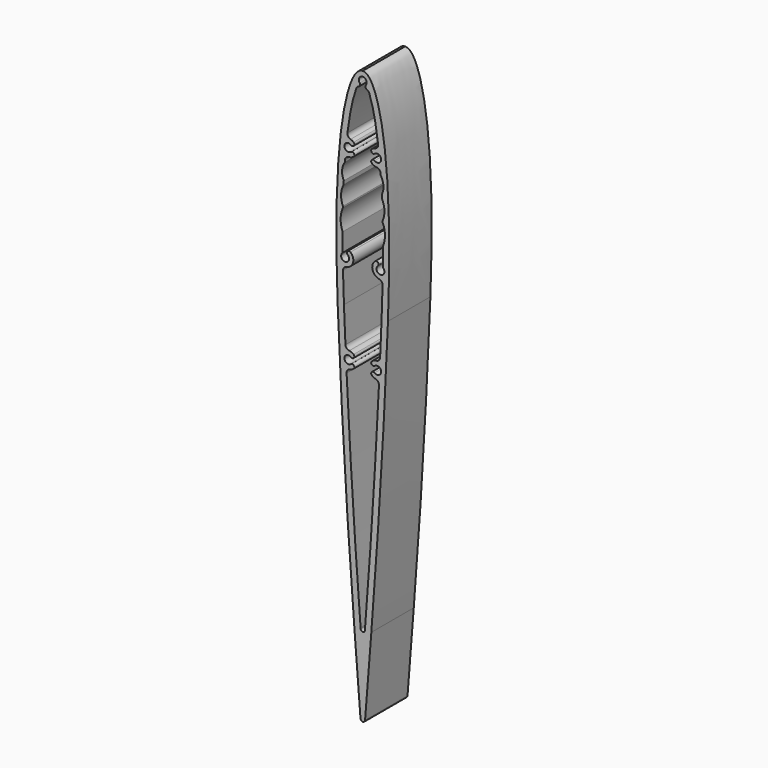
from build123d import *

# Parameters (mm, degrees)
F1_DEPTH = 25


# Not quite as in the source:
# - ends of sketch curves that miss each other by under 0.0002 mm in the source are joined
# - a feature of the source that left no trace in its solid (it failed there, or was rolled back) is left out
# - the dataset's text gives a spline's control points without its knots; the knots are read off the source's solid


with BuildPart() as f1:
    # F0 (on Front) → F1 (new body)
    with BuildSketch(Plane.XZ):
        with BuildLine():
            add(Edge.make_bspline(
                [(1.891079, 35), (1.67065, 41.443482), (1.229325, 54.34412), (1.236246, 72.62452), (1.854152, 89.816756), (2.950856, 103.206488), (4.427907, 113.848384), (5.710378, 120.445075), (7.111503, 125.630168), (8.225657, 128.804593), (9.370693, 131.232803), (10.308152, 132.76995), (11.333886, 133.94638), (12.418388, 134.799025), (13.312537, 134.933118), (13.758514, 135)],
                knots=[0, 0, 0, 0, 0.187516, 0.37543, 0.531557, 0.687815, 0.765905, 0.843992, 0.883056, 0.922083, 0.941611, 0.961119, 0.974122, 0.987093, 1, 1, 1, 1], degree=3))
            ThreePointArc((1.891079, 35), (5.18790283, -30.8265117322), (9.7346770147, -96.5785119988))
            Line((9.7346770147, -96.5785119988), (12.680055, -134.003082))
            ThreePointArc((12.680055, -134.003082), (13.758514, -135), (14.8369732342, -134.0030820184))
            Line((14.8369732342, -134.0030820184), (17.782351, -96.578512))
            ThreePointArc((17.782351, -96.578512), (22.32912517, -30.8265117322), (25.6259492802, 34.9999999886))
            add(Edge.make_bspline(
                [(25.6259492802, 34.9999999886), (25.846378, 41.443482), (26.287703, 54.34412), (26.280782, 72.62452), (25.662876, 89.816756), (24.566172, 103.206488), (23.089121, 113.848384), (21.80665, 120.445075), (20.405525, 125.630168), (19.291371, 128.804593), (18.146336, 131.232803), (17.208876, 132.76995), (16.183142, 133.94638), (15.09864, 134.799025), (14.204491, 134.933118), (13.758514, 135)],
                knots=[0, 0, 0, 0, 0.187516, 0.37543, 0.531557, 0.687815, 0.765905, 0.843992, 0.883056, 0.922083, 0.941611, 0.961119, 0.974122, 0.987093, 1, 1, 1, 1], degree=3))
        make_face()
        with BuildLine():
            ThreePointArc((10.7048396327, 126.7447711351), (11.1679770642, 127.4688001083), (11.8922270655, 127.9315918218))
            ThreePointArc((11.8922270655, 127.9315918218), (12.5128387489, 128.6095810977), (12.3178320496, 129.507802041))
            ThreePointArc((12.3178320496, 129.507802041), (13.758514, 132.57), (15.1991958566, 129.5078021187))
            ThreePointArc((15.1991958566, 129.5078021187), (15.0041892511, 128.6095810977), (15.6248008709, 127.9315916486))
            ThreePointArc((15.6248008709, 127.9315916486), (16.3490509358, 127.4688001083), (16.8121883673, 126.7447711351))
            add(Edge.make_bspline(
                [(20.994748, 106.91483), (20.92809, 107.430889), (20.443681, 111.181145), (19.486418, 116.97062), (18.068833, 123.066133), (17.103525, 125.891927), (16.8121883673, 126.7447711351)],
                knots=[0, 0, 0, 0, 0.076898, 0.558829, 0.866852, 1, 1, 1, 1], degree=3))
            ThreePointArc((20.994748, 106.91483), (20.6731029608, 105.5518093545), (19.5362950839, 104.733916692))
            ThreePointArc((19.5362950839, 104.733916692), (18.7711221159, 104.4351009548), (18.0862550366, 103.9815179558))
            ThreePointArc((18.0862550366, 103.9815179558), (17.9533759504, 102.573560959), (19.361333041, 102.4406819504))
            ThreePointArc((19.361333041, 102.4406819504), (22.423531, 100.9999996812), (19.3613326275, 99.5593185499))
            ThreePointArc((19.3613326275, 99.5593185499), (17.9533759504, 99.426440041), (18.086254959, 98.0184829504))
            ThreePointArc((18.086254959, 98.0184829504), (19.1227846437, 97.4041878714), (20.2980009563, 97.1384453394))
            ThreePointArc((20.2980009563, 97.1384453394), (21.5722847011, 96.5648538267), (22.1599911103, 95.2970180085))
            Line((22.1599911103, 95.2970180085), (22.234161, 94.316552))
            ThreePointArc((22.234161, 94.316552), (23.4953802876, 90.4894154344), (22.7148044303, 86.5361447913))
            Line((22.7148044303, 86.5361447913), (22.796247, 84.843317))
            ThreePointArc((22.796247, 84.843317), (23.9766042426, 80.3624422689), (23.1088944482, 75.8106778045))
            Line((23.1088944482, 75.8106778045), (23.123577, 75.180508))
            ThreePointArc((23.123577, 75.180508), (24.2099659037, 70.1953546002), (23.2467470629, 65.184944974))
            Line((23.2467470629, 65.184944974), (23.204994, 56.49772))
            ThreePointArc((23.204994, 56.49772), (22.1496350615, 53.1311073565), (20.8652283929, 56.4171625436))
            ThreePointArc((20.8652283929, 56.4171625436), (20.9706286801, 57.8274426551), (19.5603488793, 57.9328441402))
            ThreePointArc((19.5603488793, 57.9328441402), (18.3546280358, 53.9708929557), (21.4210798987, 51.1874254183))
            ThreePointArc((21.4210798987, 51.1874254183), (22.6231237311, 50.4867629461), (23.0773031211, 49.1716359972))
            Line((23.0773031211, 49.1716359972), (22.628414, 35.121594))
            ThreePointArc((22.628414, 35.121594), (22.2865538436, 26.9330823704), (21.9253327664, 18.7454019653))
            ThreePointArc((21.9253327664, 18.7454019653), (21.3851258225, 17.4666128328), (20.1426050047, 16.8475269564))
            ThreePointArc((20.1426050047, 16.8475269564), (19.0535819433, 16.5651685497), (18.0917870366, 15.9815179558))
            ThreePointArc((18.0917870366, 15.9815179558), (17.9589079504, 14.573560959), (19.366865041, 14.4406819504))
            ThreePointArc((19.366865041, 14.4406819504), (22.429063, 12.9999996812), (19.3668646275, 11.5593185499))
            ThreePointArc((19.3668646275, 11.5593185499), (17.9589079504, 11.426440041), (18.091786959, 10.0184829504))
            ThreePointArc((18.091786959, 10.0184829504), (18.8879332732, 9.5094090133), (19.7837219717, 9.2084638615))
            ThreePointArc((19.7837219717, 9.2084638615), (20.9627282842, 8.4756150646), (21.3806655936, 7.1518129711))
            ThreePointArc((21.3806655936, 7.1518129711), (18.4732116736, -44.6203041502), (14.7915990398, -96.3431340031))
            Line((14.7915990398, -96.3431340031), (14.755431, -96.802684))
            ThreePointArc((14.755431, -96.802684), (13.758514, -97.724225), (12.7615966608, -96.8026840267))
            Line((12.7615966608, -96.8026840267), (12.725429, -96.343134))
            ThreePointArc((12.725429, -96.343134), (9.0438163264, -44.6203041502), (6.1363623266, 7.1518129672))
            ThreePointArc((6.1363623266, 7.1518129672), (6.5542997158, 8.4756150646), (7.7333059591, 9.2084642002))
            ThreePointArc((7.7333059591, 9.2084642002), (8.6290947268, 9.5094090133), (9.4252414546, 10.0184824507))
            ThreePointArc((9.4252414546, 10.0184824507), (9.5581200496, 11.426440041), (8.150162959, 11.5593190496))
            ThreePointArc((8.150162959, 11.5593190496), (5.087965, 12.9999996812), (8.1501628813, 14.4406818566))
            ThreePointArc((8.1501628813, 14.4406818566), (9.5581200496, 14.573560959), (9.425241041, 15.9815180496))
            ThreePointArc((9.425241041, 15.9815180496), (8.4634460567, 16.5651685497), (7.3744229822, 16.8475268354))
            ThreePointArc((7.3744229822, 16.8475268354), (6.1319021775, 17.4666128328), (5.5916951118, 18.7454019598))
            ThreePointArc((5.5916951118, 18.7454019598), (5.2304741564, 26.9330823704), (4.8886135237, 35.1215939807))
            Line((4.8886135237, 35.1215939807), (4.439725, 49.171636))
            ThreePointArc((4.439725, 49.171636), (4.8939042689, 50.4867629461), (6.0959480065, 51.1874259626))
            ThreePointArc((6.0959480065, 51.1874259626), (9.1623999642, 53.9708929557), (7.9566789172, 57.9328439039))
            ThreePointArc((7.9566789172, 57.9328439039), (6.5463993199, 57.8274426551), (6.6517998105, 56.4171627799))
            ThreePointArc((6.6517998105, 56.4171627799), (5.3673929385, 53.1311073565), (4.3120343596, 56.497719519))
            Line((4.3120343596, 56.497719519), (4.270281, 65.184945))
            ThreePointArc((4.270281, 65.184945), (3.3070620963, 70.1953546002), (4.3934510499, 75.1805079779))
            Line((4.3934510499, 75.1805079779), (4.408134, 75.810678))
            ThreePointArc((4.408134, 75.810678), (3.5404237654, 80.3624424999), (4.7207818837, 84.8433170606))
            Line((4.7207818837, 84.8433170606), (4.802224, 86.536145))
            ThreePointArc((4.802224, 86.536145), (4.0216477124, 90.4894154344), (5.2828673841, 94.3165517511))
            Line((5.2828673841, 94.3165517511), (5.357037, 95.297018))
            ThreePointArc((5.357037, 95.297018), (5.9447439167, 96.5648534488), (7.2190270346, 97.1384454772))
            ThreePointArc((7.2190270346, 97.1384454772), (8.3942433563, 97.4041878714), (9.4307734546, 98.0184824507))
            ThreePointArc((9.4307734546, 98.0184824507), (9.5636520496, 99.426440041), (8.155694959, 99.5593190496))
            ThreePointArc((8.155694959, 99.5593190496), (5.093497, 100.9999996812), (8.1556948813, 102.4406818566))
            ThreePointArc((8.1556948813, 102.4406818566), (9.5636520496, 102.573560959), (9.430773041, 103.9815180496))
            ThreePointArc((9.430773041, 103.9815180496), (8.7459058841, 104.4351009548), (7.980732822, 104.7339163465))
            ThreePointArc((7.980732822, 104.7339163465), (6.8439250392, 105.5518093545), (6.5222802581, 106.9148299673))
            add(Edge.make_bspline(
                [(6.5222802581, 106.9148299673), (6.588938, 107.430889), (7.073347, 111.181145), (8.03061, 116.97062), (9.448195, 123.066133), (10.413504, 125.891927), (10.7048396327, 126.7447711351)],
                knots=[0, 0, 0, 0, 0.076898, 0.558829, 0.866852, 1, 1, 1, 1], degree=3))
        make_face(mode=Mode.SUBTRACT)
    extrude(amount=F1_DEPTH)


solid = f1.part
